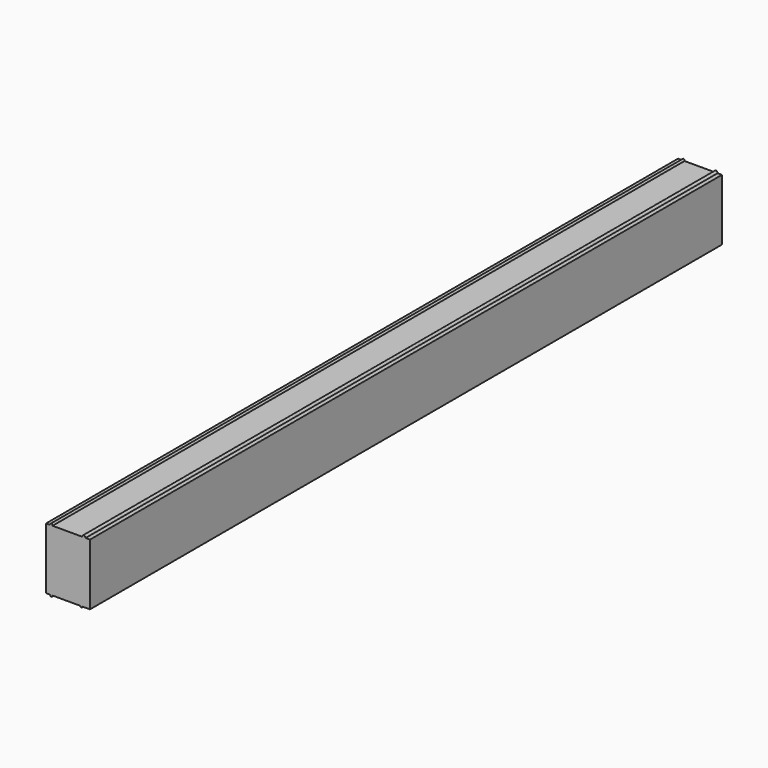
from build123d import *

# Parameters (mm, degrees)
F0_W     = 90
F0_H     = 7
F1_DEPTH = 5
F2_T     = -2
F4_DEPTH = 90
F6_DEPTH = 90
F9_DEPTH = 90


with BuildPart() as f1:
    # F0 (on Right) → F1 (new body)
    with BuildSketch(Plane.YZ):
        with Locations((13.5903862119, 3.5)):
            Rectangle(F0_W, F0_H)
    extrude(amount=F1_DEPTH)

    # F2
    f2_openings = [f1.faces().sort_by_distance(p)[0] for p in [
        (2.5, 58.590386, 3.5),
    ]]
    offset(amount=F2_T, openings=f2_openings)

    # F3 (on face) → F4 (join)
    with BuildSketch(Plane(origin=(0, 58.5903862119, 0), x_dir=(-1, 0, 0), z_dir=(0, 1, 0))):
        with BuildLine():
            add(Edge.make_bspline(
                [(-4.4927471317, 6.8335854448), (-4.5660253813, 6.9655119185), (-4.3165354389, 7.4956076145), (-3.9218503585, 6.688839741), (-4.4243988792, 6.7105346898), (-4.4927471317, 6.8335854448)],
                knots=[0, 0, 0, 0, 0.3378548186, 0.6848752994, 1, 1, 1, 1], degree=3))
        make_face()
    extrude(amount=-F4_DEPTH)

    # F5 (on face) → F6 (join)
    with BuildSketch(Plane(origin=(0, 58.5903862119, 0), x_dir=(-1, 0, 0), z_dir=(0, 1, 0))):
        with BuildLine():
            add(Edge.make_bspline(
                [(-0.7403470987, 7), (-0.744928401, 7.0852952576), (-0.61828683, 7.299312345), (-0.4655472616, 7.0863177766), (-0.4555928001, 7)],
                knots=[0.063573249, 0.063573249, 0.063573249, 0.063573249, 0.330947852, 0.5992996658, 0.5992996658, 0.5992996658, 0.5992996658], degree=3))
            Line((-0.7403470987, 7), (-0.4555928001, 7))
        make_face()
    extrude(amount=-F6_DEPTH)

    # F7 (on face) + F8 (on face) → F9 (join)
    with BuildSketch(Plane(origin=(0, 58.5903862119, 0), x_dir=(-1, 0, 0), z_dir=(0, 1, 0))):
        with BuildLine():
            Line((-0.7403470979, 0), (-0.4555928001, 0))
            add(Edge.make_bspline(
                [(-0.7403470979, 0), (-0.7018064847, 0.0647744469), (-0.4979936325, 0.0653103199), (-0.4555928001, 0)],
                knots=[0.6354416672, 0.6354416672, 0.6354416672, 0.6354416672, 1, 1, 1, 1], degree=3))
        make_face()
        with BuildLine():
            add(Edge.make_bspline(
                [(-0.4555928001, 0), (-0.4190961932, -0.0562159972), (-0.587360905, -0.2688458523), (-0.7743512153, -0.0571500481), (-0.7403470979, 0)],
                knots=[0, 0, 0, 0, 0.3137943625, 0.6354416672, 0.6354416672, 0.6354416672, 0.6354416672], degree=3))
            Line((-0.4555928001, 0), (-0.7403470979, 0))
        make_face()
    with BuildSketch(Plane(origin=(0, 58.5903862119, 0), x_dir=(-1, 0, 0), z_dir=(0, 1, 0))):
        with BuildLine():
            add(Edge.make_bspline(
                [(-3.9229183458, 0), (-3.8911392187, -0.0399748921), (-4.0049623328, -0.195717275), (-4.1958645114, -0.0440099941), (-4.1729910299, 0)],
                knots=[0, 0, 0, 0, 0.2897821962, 0.6244929237, 0.6244929237, 0.6244929237, 0.6244929237], degree=3))
            Line((-3.9229183458, 0), (-4.1729910299, 0))
        make_face()
    extrude(amount=-F9_DEPTH)


solid = f1.part
